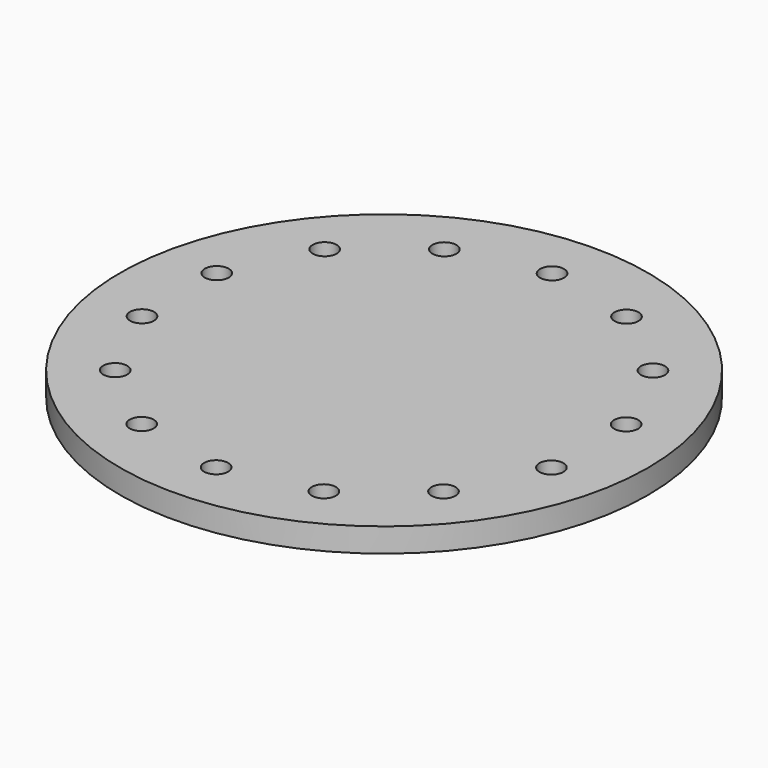
from build123d import *

# Parameters (mm, degrees)
F0_R            = 55
F1_DEPTH        = 5
F2_R            = 2.5
F3_DEPTH        = 5.001
F3_COPIES_COUNT = 14


# Not quite as in the source:
# - a pattern or mirror of a feature is missing from the dataset's text; its kind, count and spacing are read off the source's solid


with BuildPart() as f1:
    # F0 (on Top) → F1 (new body)
    with BuildSketch(Plane.XY):
        Circle(F0_R)
    extrude(amount=F1_DEPTH)

    # F2 (on face) → F3 (cut, through all)
    with BuildSketch(Plane.XY.offset(5)):
        with Locations((0, 43.75)):
            Circle(F2_R)
    f3 = extrude(amount=-F3_DEPTH, mode=Mode.SUBTRACT)

    # F3_copies: F3 ×14 about axis
    f3_copies_axis = Axis((0, 0, 0), (0, 0, 1))
    for i in range(1, F3_COPIES_COUNT):
        add(f3.rotate(f3_copies_axis, i * 360 / F3_COPIES_COUNT), mode=Mode.SUBTRACT)


solid = f1.part
